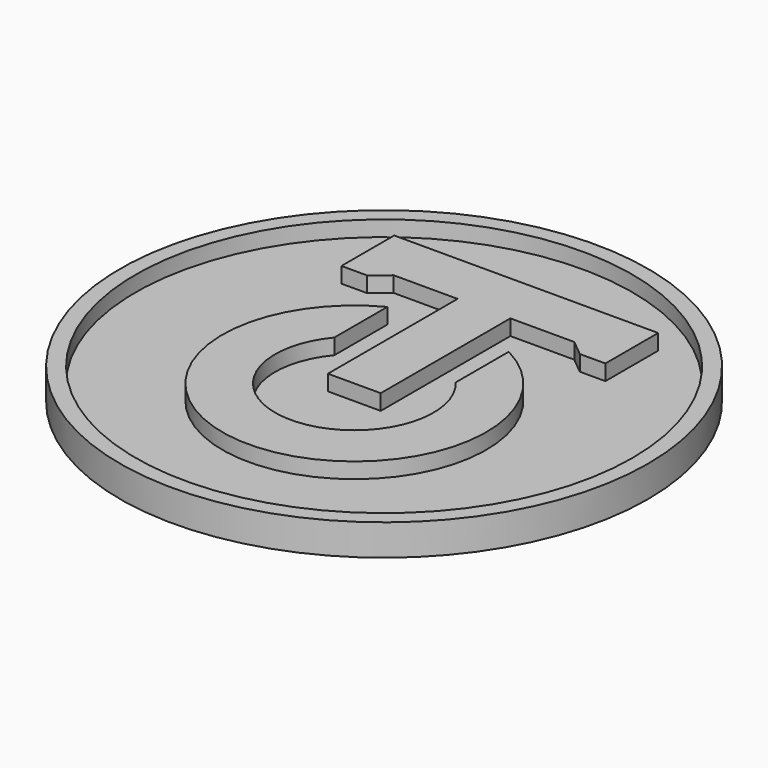
from build123d import *

# Parameters (mm, degrees)
F0_R         = 25.4
F1_DEPTH     = 1.5
F2_R         = 25.4
F2_R_2       = 23.9
F3_DEPTH     = 1.5
F5_DEPTH     = 1.5
F6_TEXT_SIZE = 17.6388888889
F7_DEPTH     = 0.6


# Not quite as in the source:
# - Text() gives the source's letters only with a copy of the font that has no kerning and outlines rounded to 1/6400 em; it was checked with that copy


with BuildPart() as f1:
    # F0 (on Top) → F1 (new body)
    with BuildSketch(Plane.XY):
        Circle(F0_R)
    extrude(amount=F1_DEPTH)

    # F2 (on face) → F3 (join)
    with BuildSketch(Plane.XY.offset(1.5)):
        Circle(F2_R)
        Circle(F2_R_2, mode=Mode.SUBTRACT)
    extrude(amount=F3_DEPTH)

    # F4 (on face) → F5 (join)
    with BuildSketch(Plane.XY.offset(1.5)):
        with BuildLine():
            Line((-5.842, 1.3123855122), (-5.842, 7.6965702233))
            ThreePointArc((-5.842, 7.6965702233), (0, -16.28), (5.842, 7.6965702233))
            Line((5.842, 7.6965702233), (5.842, 1.3123855122))
            ThreePointArc((5.842, 1.3123855122), (0, -11.2), (-5.842, 1.3123855122))
        make_face()
        Polygon((-2.54, -3.58), (0, -3.58), (2.54, -3.58), (2.54, 12.0138577503), (8.6917923763, 12.0138577503), (10.2369999513, 10.7438577503), (12.7, 10.7438577503), (12.7, 17.0938577503), (0, 17.0938577503), (-12.7, 17.0938577503), (-12.7, 10.7438577503), (-10.2369999513, 10.7438577503), (-8.6917923763, 12.0138577503), (-2.54, 12.0138577503), align=None)
    extrude(amount=F5_DEPTH)

    # F6 (on face) → F7 (cut)
    with BuildSketch(Plane(origin=(0, 0, 0), x_dir=(1, 0, 0), z_dir=(0, 0, -1))):
        with Locations(Location((19.7955186632, 6.35), (0, 0, 180))):
            Text('2543', F6_TEXT_SIZE, font='Open Sans', font_style=FontStyle.BOLD, text_align=(TextAlign.LEFT, TextAlign.BOTTOM))
    extrude(amount=-F7_DEPTH, mode=Mode.SUBTRACT)


solid = f1.part
